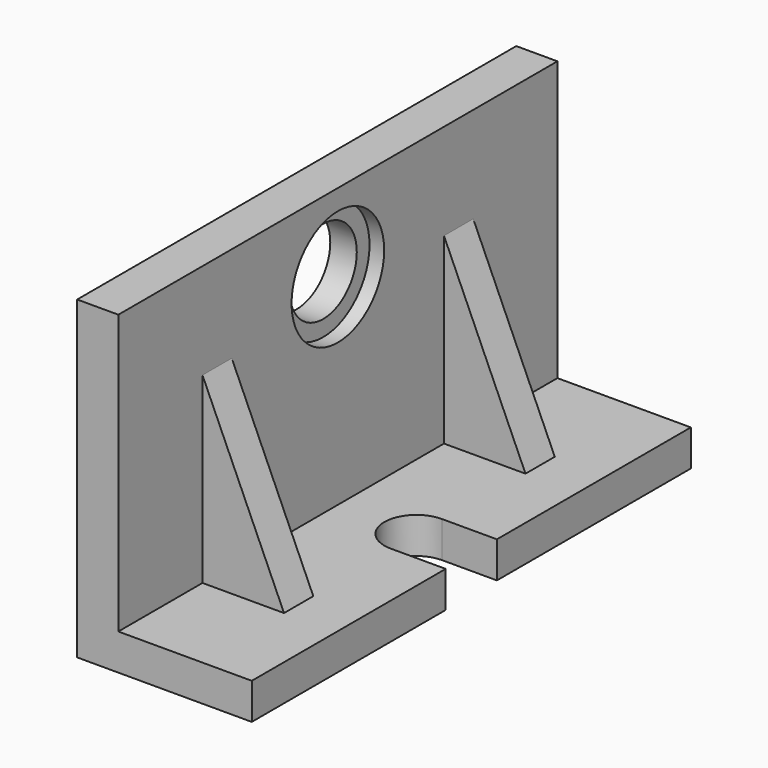
from build123d import *

# Parameters (mm, degrees)
F1_DEPTH  = 76.2
F2_R      = 11.6445519737
F3_DEPTH  = 12.7
F4_R      = 16.0689830222
F4_R_2    = 11.6445519737
F5_DEPTH  = 4.064
F7_DEPTH  = 10.0515203009
F10_DEPTH = 10.16


# Not quite as in the source:
# - a pattern or mirror of a feature is missing from the dataset's text; its kind, count and spacing are read off the source's solid


with BuildPart() as f1:
    # F0 (on Front) → F1 (new body, symmetric)
    with BuildSketch(Plane.XZ):
        Polygon((-46.9024144113, -27.3925848305), (-46.9024144113, 50.0555187464), (-58.332413435, 50.0555187464), (-58.332413435, -37.4431051314), (-9.8534487188, -37.4431051314), (-9.8534487188, -27.3925848305), align=None)
    extrude(amount=F1_DEPTH, both=True)

    # F2 (on face) → F3 (cut, symmetric)
    with BuildSketch(Plane.YZ.offset(-46.9024144113)):
        with Locations((0, 28.3396150917)):
            Circle(F2_R)
    extrude(amount=F3_DEPTH, both=True, mode=Mode.SUBTRACT)

    # F4 (on face) → F5 (cut)
    with BuildSketch(Plane.YZ.offset(-46.9024144113)):
        with Locations((0, 28.3396150917)):
            Circle(F4_R)
        with Locations((0, 28.3396150917)):
            Circle(F4_R_2, mode=Mode.SUBTRACT)
    extrude(amount=-F5_DEPTH, mode=Mode.SUBTRACT)

    # F6 (on face) → F7 (cut, through all)
    with BuildSketch(Plane.XY.offset(-27.3925848305)):
        with BuildLine():
            ThreePointArc((-25.0934487188, -8.89), (-18.807269434, -6.2861792847), (-16.2034487188, 0))
            ThreePointArc((-16.2034487188, 0), (-18.807269434, 6.2861792847), (-25.0934487188, 8.89))
            ThreePointArc((-25.0934487188, 8.89), (-33.9834487188, 0), (-25.0934487188, -8.89))
        make_face()
        with BuildLine():
            ThreePointArc((-25.0934487188, 8.89), (-18.807269434, 6.2861792847), (-16.2034487188, 0))
            ThreePointArc((-16.2034487188, 0), (-18.807269434, -6.2861792847), (-25.0934487188, -8.89))
            Line((-25.0934487188, -8.89), (-9.8534487188, -8.89))
            Line((-9.8534487188, -8.89), (-9.8534487188, 8.89))
            Line((-9.8534487188, 8.89), (-25.0934487188, 8.89))
        make_face()
    extrude(amount=-F7_DEPTH, mode=Mode.SUBTRACT)

    # F9 (on offset) → F10 (join)
    with BuildSketch(Plane.XZ.offset(-46.99)):
        Polygon((-24.2647007108, -27.3925848305), (-46.9024144113, 23.4074151695), (-46.9024144113, -27.3925848305), align=None)
    f10 = extrude(amount=F10_DEPTH)

    # F10_copies: F10 across plane
    add(f10.mirror(Plane(origin=(0, 0, 0), x_dir=(0, 0, -1), z_dir=(0, -1, 0))))


solid = f1.part
